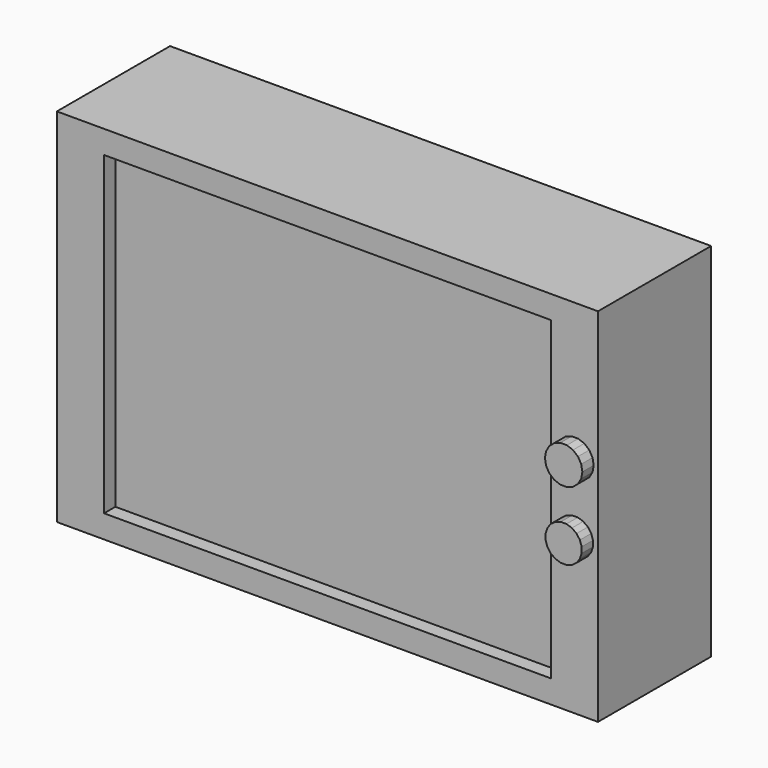
from build123d import *

# Parameters (mm, degrees)
F0_W     = 80.216743052
F0_H     = 56.6479042172
F1_DEPTH = 25.4
F2_DEPTH = 22.86
F3_DEPTH = 27.94
F4_DEPTH = 27.94


# Not quite as in the source:
# - the program builds the solid bodies; features that only make, move or delete a surface that nothing else refers to are left out


with BuildPart() as f1:
    # F0 (on Front) → F1 (new body)
    with BuildSketch(Plane.XZ):
        Polygon((-48.5848858953, 32.4588380754), (-48.5848858953, -32.4588380754), (48.5848858953, -32.4588380754), (48.5848858953, 32.4588380754), (23.2139006257, 32.4588380754), align=None)
        Polygon((45.9382493502, -7.469226185), (44.9628157303, -7.7861637805), (43.9371841267, -7.7861637805), (42.9617505067, -7.469226185), (42.1319971095, -6.8663750542), (41.5291459786, -6.0366216569), (41.2122083831, -5.061188037), (41.2122083831, -4.0355564333), (41.5291459786, -3.0601228134), (42.1319971095, -2.2303694161), (42.9617505067, -1.6275182853), (43.9371841267, -1.3105806898), (44.9628157303, -1.3105806898), (45.9382493502, -1.6275182853), (46.7680027475, -2.2303694161), (47.3708538784, -3.0601228134), (47.6877914738, -4.0355564333), (47.6877914738, -5.061188037), (47.3708538784, -6.0366216569), (46.7680027475, -6.8663750542), align=None, mode=Mode.SUBTRACT)
        Rectangle(F0_W, F0_H, mode=Mode.SUBTRACT)
        Polygon((46.129602097, 4.9471233192), (45.03331964, 4.5481091365), (43.8666802169, 4.5481091365), (42.77039776, 4.9471233192), (41.8767001128, 5.6970246853), (41.2933804012, 6.7073640628), (41.0907955914, 7.8562796116), (41.2933804012, 9.0051951604), (41.8767001128, 10.0155345378), (42.77039776, 10.765435904), (43.8666802169, 11.1644500867), (45.03331964, 11.1644500867), (46.129602097, 10.765435904), (47.0232997442, 10.0155345378), (47.6066194557, 9.0051951604), (47.8092042655, 7.8562796116), (47.6066194557, 6.7073640628), (47.0232997442, 5.6970246853), align=None, mode=Mode.SUBTRACT)
    extrude(amount=F1_DEPTH)

    # F0 (on Front) → F2 (join)
    with BuildSketch(Plane.XZ):
        Rectangle(F0_W, F0_H)
    extrude(amount=F2_DEPTH)

    # F0 (on Front) → F3 (join)
    with BuildSketch(Plane.XZ):
        Polygon((43.8666802169, 4.5481091365), (45.03331964, 4.5481091365), (46.129602097, 4.9471233192), (47.0232997442, 5.6970246853), (47.6066194557, 6.7073640628), (47.8092042655, 7.8562796116), (47.6066194557, 9.0051951604), (47.0232997442, 10.0155345378), (46.129602097, 10.765435904), (45.03331964, 11.1644500867), (43.8666802169, 11.1644500867), (42.77039776, 10.765435904), (41.8767001128, 10.0155345378), (41.2933804012, 9.0051951604), (41.0907955914, 7.8562796116), (41.2933804012, 6.7073640628), (41.8767001128, 5.6970246853), (42.77039776, 4.9471233192), align=None)
    extrude(amount=F3_DEPTH)

    # F0 (on Front) → F4 (join)
    with BuildSketch(Plane.XZ):
        Polygon((43.9371841267, -7.7861637805), (44.9628157303, -7.7861637805), (45.9382493502, -7.469226185), (46.7680027475, -6.8663750542), (47.3708538784, -6.0366216569), (47.6877914738, -5.061188037), (47.6877914738, -4.0355564333), (47.3708538784, -3.0601228134), (46.7680027475, -2.2303694161), (45.9382493502, -1.6275182853), (44.9628157303, -1.3105806898), (43.9371841267, -1.3105806898), (42.9617505067, -1.6275182853), (42.1319971095, -2.2303694161), (41.5291459786, -3.0601228134), (41.2122083831, -4.0355564333), (41.2122083831, -5.061188037), (41.5291459786, -6.0366216569), (42.1319971095, -6.8663750542), (42.9617505067, -7.469226185), align=None)
    extrude(amount=F4_DEPTH)


solid = f1.part
